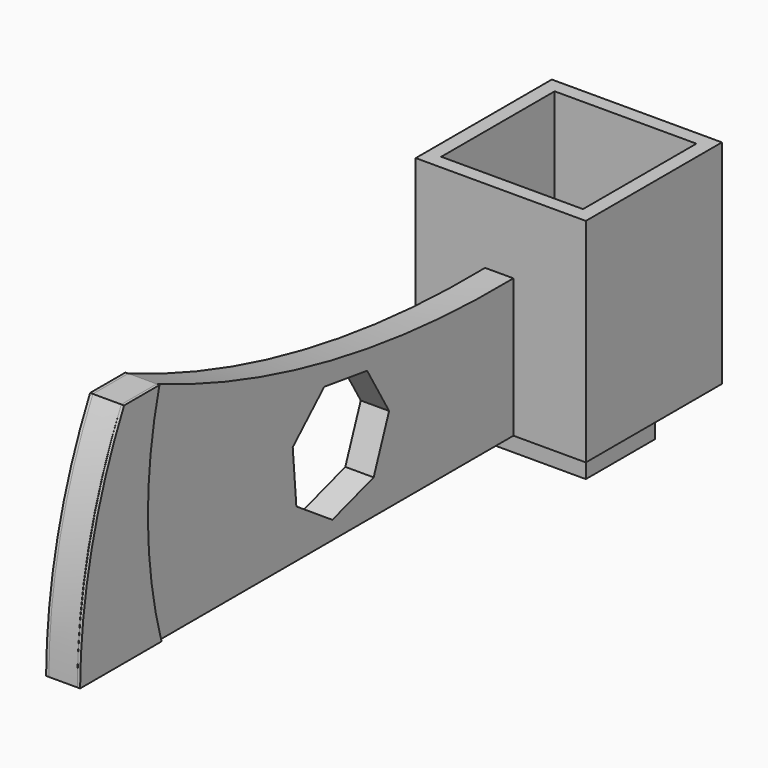
from build123d import *

# Parameters (mm, degrees)
F0_W      = 30.48
F0_H      = 30.48
F1_DEPTH  = 19.05
F2_W      = 18.5134310317
F2_H      = 15.5255280393
F3_DEPTH  = 7.62
F5_DEPTH  = 21.59
F6_W      = 97.6882427931
F6_H      = 2.54
F7_DEPTH  = 25.4
F9_DEPTH  = 25.4
F11_DEPTH = 0.508
F13_DEPTH = 0.508
F15_DEPTH = 25.4
F16_W     = 25.4
F16_H     = 25.4
F17_DEPTH = 25.4


with BuildPart() as f1:
    # F0 (on Top) → F1 (new body, symmetric)
    with BuildSketch(Plane.XY):
        with Locations((15.24, 15.24)):
            Rectangle(F0_W, F0_H)
    extrude(amount=F1_DEPTH, both=True)

    # F2 (on face) → F3 (join)
    with BuildSketch(Plane(origin=(0, 0, -19.05), x_dir=(1, 0, 0), z_dir=(0, 0, -1))):
        with Locations((15.24, -15.24)):
            Rectangle(F2_W, F2_H)
    extrude(amount=F3_DEPTH)

    # F4 (on Top) → F5 (join, symmetric)
    with BuildSketch(Plane.XY):
        Polygon((17.506013127, 0), (12.426013127, 0), (12.426013127, -97.6882427931), (14.966013127, -97.6882427931), (17.506013127, -97.6882427931), align=None)
    extrude(amount=F5_DEPTH, both=True)

    # F6 (on face) → F7 (cut)
    with BuildSketch(Plane.YZ.offset(17.506013127)):
        with BuildLine():
            ThreePointArc((-79.9160450697, 21.59), (-40.8055075971, 9.3997324049), (0, 5.7738097385))
            Line((0, 5.7738097385), (0, 9.3484056997))
            Line((0, 9.3484056997), (0, 19.05))
            Line((0, 19.05), (0, 21.59))
            Line((0, 21.59), (-67.3900023103, 21.59))
            Line((-67.3900023103, 21.59), (-79.9160450697, 21.59))
        make_face()
        with Locations((-48.8441213965, -20.32)):
            Rectangle(F6_W, F6_H)
    extrude(amount=-F7_DEPTH, mode=Mode.SUBTRACT)

    # F8 (on face) → F9 (cut)
    with BuildSketch(Plane.YZ.offset(17.506013127)):
        with BuildLine():
            ThreePointArc((-97.6882427931, -19.05), (-95.1897163869, 1.8587252761), (-87.8348387778, 21.59))
            Line((-87.8348387778, 21.59), (-97.6882427931, 21.59))
            Line((-97.6882427931, 21.59), (-97.6882427931, -19.05))
        make_face()
    extrude(amount=-F9_DEPTH, mode=Mode.SUBTRACT)

    # F14 (on face) → F15 (cut)
    with BuildSketch(Plane.YZ.offset(18.014013127)):
        Polygon((-31.3068207463, -12.8963272836), (-27.8436254601, -3.8319919441), (-32.7711412533, 4.5271638053), (-42.3788482306, 5.8865251898), (-49.4319470766, -0.7775346392), (-48.6193105033, -10.4468427083), (-40.5528704251, -15.8402128236), align=None)
    extrude(amount=-F15_DEPTH, mode=Mode.SUBTRACT)

    # F16 (on face) → F17 (cut)
    with BuildSketch(Plane.XY.offset(19.05)):
        with Locations((15.24, 15.24)):
            Rectangle(F16_W, F16_H)
    extrude(amount=-F17_DEPTH, mode=Mode.SUBTRACT)


with BuildPart() as f11:
    # F10 (on face) → F11 (new body)
    with BuildSketch(Plane.YZ.offset(17.506013127)):
        with BuildLine():
            ThreePointArc((-79.454369843, -19.05), (-82.4983241821, 1.2380426599), (-79.9160450697, 21.59))
            Line((-79.9160450697, 21.59), (-87.8348387778, 21.59))
            ThreePointArc((-87.8348387778, 21.59), (-95.1158094508, 1.8408061102), (-97.6882427931, -19.05))
            Line((-97.6882427931, -19.05), (-79.454369843, -19.05))
        make_face()
    extrude(amount=F11_DEPTH)


with BuildPart() as f13:
    # F12 (on face) → F13 (new body)
    with BuildSketch(Plane(origin=(12.426013127, 0, 0), x_dir=(0, -1, 0), z_dir=(-1, 0, 0))):
        with BuildLine():
            Line((87.8348387778, 21.59), (79.9160450697, 21.59))
            ThreePointArc((79.9160450697, 21.59), (82.4983241821, 1.2380426599), (79.454369843, -19.05))
            Line((79.454369843, -19.05), (97.6882427931, -19.05))
            ThreePointArc((97.6882427931, -19.05), (95.1146199968, 1.8405177202), (87.8348387778, 21.59))
        make_face()
        with BuildLine():
            ThreePointArc((79.454369843, -19.05), (82.4983241821, 1.2380426599), (79.9160450697, 21.59))
            ThreePointArc((79.9160450697, 21.59), (82.3436895998, 1.2397993271), (79.454369843, -19.05))
        make_face()
        with BuildLine():
            ThreePointArc((97.6882427931, -19.05), (95.1158094508, 1.8408061102), (87.8348387778, 21.59))
            ThreePointArc((87.8348387778, 21.59), (95.1146199968, 1.8405177202), (97.6882427931, -19.05))
        make_face()
    extrude(amount=F13_DEPTH)


solid = Compound([f1.part, f11.part, f13.part])
